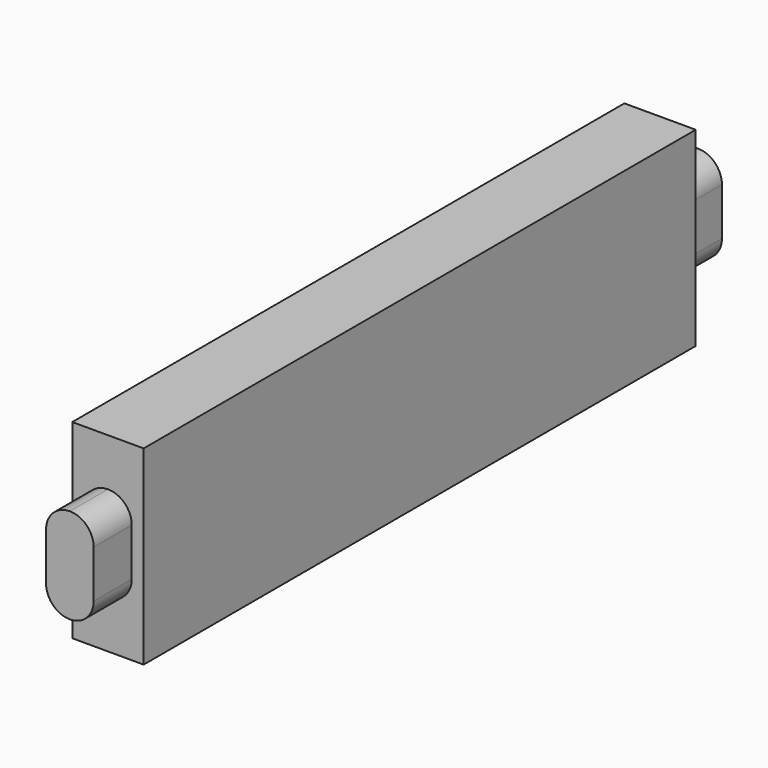
from build123d import *

# Parameters (mm, degrees)
F0_W     = 19.05
F0_H     = 184.15
F1_DEPTH = 50.8
F2_W     = 12.7
F2_H     = 25.4
F3_DEPTH = 12.7
F4_W     = 12.7
F4_H     = 25.4
F5_DEPTH = 12.7
F6_R     = 6.34999


# Not quite as in the source:
# - a fillet or chamfer is up to 0.001 mm smaller than in the source, because OpenCascade refuses the exact size


with BuildPart() as f1:
    # F0 (on Top) → F1 (new body)
    with BuildSketch(Plane.XY):
        Rectangle(F0_W, F0_H)
    extrude(amount=-F1_DEPTH)

    # F2 (on face) → F3 (join)
    with BuildSketch(Plane.XZ.offset(92.075)):
        with Locations((0, -25.4)):
            Rectangle(F2_W, F2_H)
    extrude(amount=F3_DEPTH)

    # F4 (on face) → F5 (join)
    with BuildSketch(Plane(origin=(0, 92.075, 0), x_dir=(-1, 0, 0), z_dir=(0, 1, 0))):
        with Locations((0, -25.4)):
            Rectangle(F4_W, F4_H)
    extrude(amount=F5_DEPTH)

    # F6 (radius 6.35 in the source; OpenCascade refuses exactly that, so slightly less here)
    f6_edges = [f1.edges().sort_by_distance(p)[0] for p in [
        (6.35, 98.425, -12.7),
        (-6.35, 98.425, -12.7),
        (-6.35, 98.425, -38.1),
        (6.35, 98.425, -38.1),
        (-6.35, -98.425, -12.7),
        (6.35, -98.425, -12.7),
        (-6.35, -98.425, -38.1),
        (6.35, -98.425, -38.1),
    ]]
    fillet(f6_edges, radius=F6_R)


solid = f1.part
